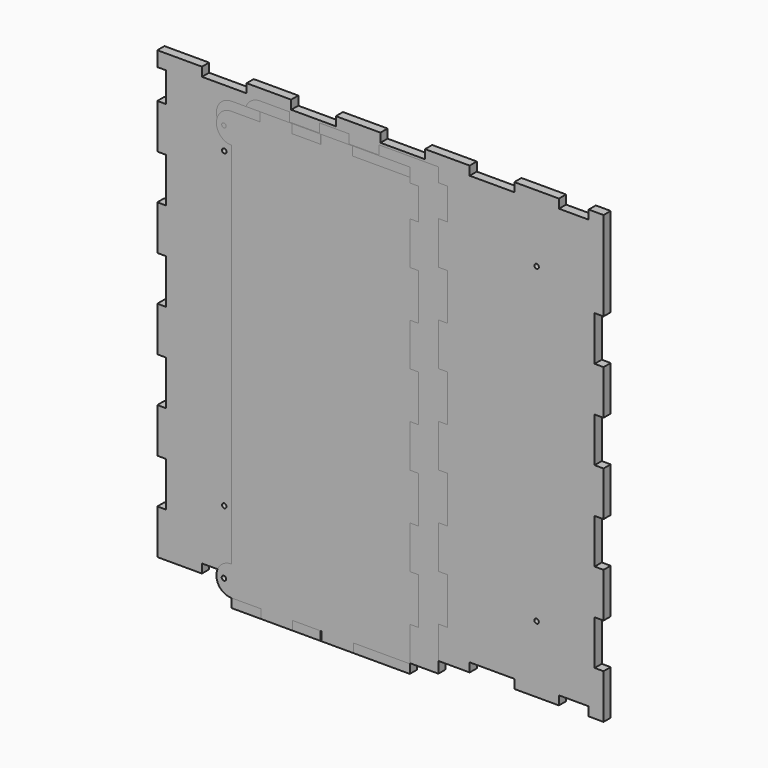
from build123d import *

# Parameters (mm, degrees)
F0_R     = 0.75
F4_DEPTH = 3
F1_R     = 0.75
F5_DEPTH = 3
F2_R     = 0.75
F6_DEPTH = 3
F3_R     = 0.75
F7_DEPTH = 3


# Not quite as in the source:
# - ends of sketch curves that miss each other by under 0.0002 mm in the source are joined


with BuildPart() as f4:
    # F0 (on Front) → F4 (new body)
    with BuildSketch(Plane.XZ):
        Polygon((-45, 72), (-60, 72), (-60, 75), (-72.0000029802, 75), (-75, 75), (-75.0000029802, 70), (-72.0000029802, 70), (-72.0000029802, 60), (-75.0000029802, 60), (-75.0000029802, 45), (-72.0000029802, 45), (-72.0000029802, 30), (-75.0000029802, 30), (-75.0000029802, 15), (-72.0000029802, 15), (-72.0000029802, 0), (-75.0000029802, 0), (-75.0000029802, -15), (-72.0000029802, -15), (-72.0000029802, -30), (-75.0000029802, -30), (-75.0000029802, -45), (-72.0000029802, -45), (-72.0000029802, -60), (-75.0000029802, -60), (-75.0000029802, -75), (-72.0000029802, -75), (-60, -75), (-60, -72), (-45, -72), (-45, -75), (-30, -75), (-30, -72), (-15, -72), (-15, -75), (0, -75), (0, -72), (15, -72), (15, -75), (30, -75), (30, -72), (45, -72), (45, -75), (60, -75), (60, -72), (70, -72), (70, -75), (75, -75), (75, -72.0000029802), (75, -60), (72, -60), (72, -45), (75, -45), (75, -30), (72, -30), (72, -15), (75, -15), (75, 0), (72, 0), (72, 15), (75, 15), (75, 30), (72, 30), (72, 45), (75, 45), (75, 60), (75, 70.000000298), (75, 75.000000298), (70, 75), (70, 72), (60, 72), (60, 75), (45, 75), (45, 72), (30, 72), (30, 75), (15, 75), (15, 72), (0, 72), (0, 75), (-15, 75), (-15, 72), (-30, 72), (-30, 75), (-45, 75), align=None)
        with Locations((-52.5, -52.5)):
            Circle(F0_R, mode=Mode.SUBTRACT)
        with Locations((52.5, -52.5)):
            Circle(F0_R, mode=Mode.SUBTRACT)
        with Locations((-52.5, 52.5)):
            Circle(F0_R, mode=Mode.SUBTRACT)
        with Locations((52.5, 52.5)):
            Circle(F0_R, mode=Mode.SUBTRACT)
    extrude(amount=F4_DEPTH)


with BuildPart() as f5:
    # F1 (on Front) → F5 (new body)
    with BuildSketch(Plane.XZ):
        with BuildLine():
            Line((22.4781758341, -64.0899424732), (22.4781758341, -63.7899424732))
            Line((22.4781758341, -63.7899424732), (22.4781758341, -48.7899424732))
            Line((22.4781758341, -48.7899424732), (22.4781758341, -48.4899424732))
            Line((22.4781758341, -48.4899424732), (19.4781758341, -48.4899424732))
            Line((19.4781758341, -48.4899424732), (19.4781758341, -34.0899424732))
            Line((19.4781758341, -34.0899424732), (22.4781758341, -34.0899424732))
            Line((22.4781758341, -34.0899424732), (22.4781758341, -33.7899424732))
            Line((22.4781758341, -33.7899424732), (22.4781758341, -18.7899424732))
            Line((22.4781758341, -18.7899424732), (22.4781758341, -18.4899424732))
            Line((22.4781758341, -18.4899424732), (19.4781758341, -18.4899424732))
            Line((19.4781758341, -18.4899424732), (19.4781758341, -4.0899424732))
            Line((19.4781758341, -4.0899424732), (22.4781758341, -4.0899424732))
            Line((22.4781758341, -4.0899424732), (22.4781758341, -3.7899424732))
            Line((22.4781758341, -3.7899424732), (22.4781758341, 11.2100575268))
            Line((22.4781758341, 11.2100575268), (22.4781758341, 11.5100575268))
            Line((22.4781758341, 11.5100575268), (19.4781758341, 11.5100575268))
            Line((19.4781758341, 11.5100575268), (19.4781758341, 25.9100575268))
            Line((19.4781758341, 25.9100575268), (22.4781758341, 25.9100575268))
            Line((22.4781758341, 25.9100575268), (22.4781758341, 26.2100575268))
            Line((22.4781758341, 26.2100575268), (22.4781758341, 41.2100575268))
            Line((22.4781758341, 41.2100575268), (22.4781758341, 41.5100575268))
            Line((22.4781758341, 41.5100575268), (19.4781758341, 41.5100575268))
            Line((19.4781758341, 41.5100575268), (19.4781758341, 55.9100575268))
            Line((19.4781758341, 55.9100575268), (22.4781758341, 55.9100567043))
            Line((22.4781758341, 55.9100567043), (22.4781758341, 56.2100567043))
            Line((22.4781758341, 56.2100567043), (22.4781758341, 66.2100567043))
            Line((22.4781758341, 66.2100567043), (22.4781758341, 66.5100567043))
            Line((22.4781758341, 66.5100567043), (19.4781758341, 66.5100567043))
            Line((19.4781758341, 66.5100567043), (19.4781758341, 71.2100575268))
            Line((19.4781758341, 71.2100575268), (-0.5218241659, 71.2100575268))
            Line((-0.5218241659, 71.2100575268), (-0.5218241659, 68.2100575268))
            Line((-0.5218241659, 68.2100575268), (-10.5218241659, 68.2100575268))
            Line((-10.5218241659, 68.2100575268), (-10.5218241659, 71.2100575268))
            Line((-10.5218241659, 71.2100575268), (-20.5218241659, 71.2100575268))
            Line((-20.5218241659, 71.2100575268), (-20.5218241659, 68.2100575268))
            Line((-20.5218241659, 68.2100575268), (-30.5218241659, 68.2100575268))
            Line((-30.5218241659, 68.2100575268), (-30.5218241659, 71.2100575268))
            Line((-30.5218241659, 71.2100575268), (-40.5218241659, 71.2100575268))
            ThreePointArc((-40.5218241659, 71.2100575268), (-45.5331626093, 66.1987190834), (-40.5218241659, 61.18738064))
            Line((-40.5218241659, 61.18738064), (-40.5218241659, -78.7899424732))
            Line((-40.5218241659, -78.7899424732), (-30.5218238408, -78.7899424732))
            Line((-30.5218238408, -78.7899424732), (-30.5218238408, -75.7899424732))
            Line((-30.5218238408, -75.7899424732), (-20.5218238408, -75.7899424732))
            Line((-20.5218238408, -75.7899424732), (-20.5218238408, -78.7899424732))
            Line((-20.5218238408, -78.7899424732), (-10.5218238408, -78.7899424732))
            Line((-10.5218238408, -78.7899424732), (-10.5218238408, -75.7899424732))
            Line((-10.5218238408, -75.7899424732), (-0.5218238408, -75.7899424732))
            Line((-0.5218238408, -75.7899424732), (-0.5218238408, -78.7899424732))
            Line((-0.5218238408, -78.7899424732), (19.4781761592, -78.7899424732))
            Line((19.4781761592, -78.7899424732), (19.4781758341, -64.0899424732))
            Line((19.4781758341, -64.0899424732), (22.4781758341, -64.0899424732))
        make_face()
        with Locations((-43.0020329712, 66.1973134672)):
            Circle(F1_R, mode=Mode.SUBTRACT)
    extrude(amount=F5_DEPTH)


with BuildPart() as f6:
    # F2 (on Front) → F6 (new body)
    with BuildSketch(Plane.XZ):
        with BuildLine():
            Line((12.8783458498, -67.2765442915), (12.8783458498, -66.9765442915))
            Line((12.8783458498, -66.9765442915), (12.8783458498, -51.9765442915))
            Line((12.8783458498, -51.9765442915), (12.8783458498, -51.6765442915))
            Line((12.8783458498, -51.6765442915), (9.8783458498, -51.6765442915))
            Line((9.8783458498, -51.6765442915), (9.8783458498, -37.2765442915))
            Line((9.8783458498, -37.2765442915), (12.8783458498, -37.2765442915))
            Line((12.8783458498, -37.2765442915), (12.8783458498, -36.9765442915))
            Line((12.8783458498, -36.9765442915), (12.8783458498, -21.9765442915))
            Line((12.8783458498, -21.9765442915), (12.8783458498, -21.6765442915))
            Line((12.8783458498, -21.6765442915), (9.8783458498, -21.6765442915))
            Line((9.8783458498, -21.6765442915), (9.8783458498, -7.2765442915))
            Line((9.8783458498, -7.2765442915), (12.8783458498, -7.2765442915))
            Line((12.8783458498, -7.2765442915), (12.8783458498, -6.9765442915))
            Line((12.8783458498, -6.9765442915), (12.8783458498, 8.0234557085))
            Line((12.8783458498, 8.0234557085), (12.8783458498, 8.3234557085))
            Line((12.8783458498, 8.3234557085), (9.8783458498, 8.3234557085))
            Line((9.8783458498, 8.3234557085), (9.8783458498, 22.7234557085))
            Line((9.8783458498, 22.7234557085), (12.8783458498, 22.7234557085))
            Line((12.8783458498, 22.7234557085), (12.8783458498, 23.0234557085))
            Line((12.8783458498, 23.0234557085), (12.8783458498, 38.0234557085))
            Line((12.8783458498, 38.0234557085), (12.8783458498, 38.3234557085))
            Line((12.8783458498, 38.3234557085), (9.8783458498, 38.3234557085))
            Line((9.8783458498, 38.3234557085), (9.8783458498, 52.7234557085))
            Line((9.8783458498, 52.7234557085), (9.8783458498, 63.3234557085))
            Line((9.8783458498, 63.3234557085), (9.8783458498, 68.0234557085))
            Line((9.8783458498, 68.0234557085), (-10.1216541502, 68.0234557085))
            Line((-10.1216541502, 68.0234557085), (-10.1216541502, 65.0234557085))
            Line((-10.1216541502, 65.0234557085), (-20.1216541502, 65.0234557085))
            Line((-20.1216541502, 65.0234557085), (-20.1216541502, 68.0234557085))
            Line((-20.1216541502, 68.0234557085), (-30.1216541502, 68.0234557085))
            Line((-30.1216541502, 68.0234557085), (-30.1216541502, 65.0234557085))
            Line((-30.1216541502, 65.0234557085), (-40.1216541502, 65.0234557085))
            Line((-40.1216541502, 65.0234557085), (-40.1216541502, 68.0234557085))
            Line((-40.1216541502, 68.0234557085), (-50.1216541502, 68.0234557085))
            ThreePointArc((-50.1216541502, 68.0234557085), (-55.1329925936, 63.0121172651), (-50.1216541502, 58.0007788217))
            Line((-50.1216541502, 58.0007788217), (-50.1216541502, -81.9765442915))
            Line((-50.1216541502, -81.9765442915), (-40.121653825, -81.9765442915))
            Line((-40.121653825, -81.9765442915), (-40.121653825, -78.9765442915))
            Line((-40.121653825, -78.9765442915), (-30.121653825, -78.9765442915))
            Line((-30.121653825, -78.9765442915), (-30.121653825, -81.9765442915))
            Line((-30.121653825, -81.9765442915), (-20.121653825, -81.9765442915))
            Line((-20.121653825, -81.9765442915), (-20.121653825, -78.9765442915))
            Line((-20.121653825, -78.9765442915), (-10.121653825, -78.9765442915))
            Line((-10.121653825, -78.9765442915), (-10.121653825, -81.9765442915))
            Line((-10.121653825, -81.9765442915), (9.878346175, -81.9765442915))
            Line((9.878346175, -81.9765442915), (9.8783458498, -67.2765442915))
            Line((9.8783458498, -67.2765442915), (12.8783458498, -67.2765442915))
        make_face()
        with Locations((-52.6018629554, 63.0107116489)):
            Circle(F2_R, mode=Mode.SUBTRACT)
    extrude(amount=F6_DEPTH)


with BuildPart() as f7:
    # F3 (on Front) → F7 (new body)
    with BuildSketch(Plane.XZ):
        with BuildLine():
            Line((12.8783458498, -67.2765442915), (12.8783458498, -66.9765442915))
            Line((12.8783458498, -66.9765442915), (12.8783458498, -51.9765442915))
            Line((12.8783458498, -51.9765442915), (12.8783458498, -51.6765442915))
            Line((12.8783458498, -51.6765442915), (9.8783458498, -51.6765442915))
            Line((9.8783458498, -51.6765442915), (9.8783458498, -37.2765442915))
            Line((9.8783458498, -37.2765442915), (12.8783458498, -37.2765442915))
            Line((12.8783458498, -37.2765442915), (12.8783458498, -36.9765442915))
            Line((12.8783458498, -36.9765442915), (12.8783458498, -21.9765442915))
            Line((12.8783458498, -21.9765442915), (12.8783458498, -21.6765442915))
            Line((12.8783458498, -21.6765442915), (9.8783458498, -21.6765442915))
            Line((9.8783458498, -21.6765442915), (9.8783458498, -7.2765442915))
            Line((9.8783458498, -7.2765442915), (12.8783458498, -7.2765442915))
            Line((12.8783458498, -7.2765442915), (12.8783458498, -6.9765442915))
            Line((12.8783458498, -6.9765442915), (12.8783458498, 8.0234557085))
            Line((12.8783458498, 8.0234557085), (12.8783458498, 8.3234557085))
            Line((12.8783458498, 8.3234557085), (9.8783458498, 8.3234557085))
            Line((9.8783458498, 8.3234557085), (9.8783458498, 22.7234557085))
            Line((9.8783458498, 22.7234557085), (12.8783458498, 22.7234557085))
            Line((12.8783458498, 22.7234557085), (12.8783458498, 23.0234557085))
            Line((12.8783458498, 23.0234557085), (12.8783458498, 38.0234557085))
            Line((12.8783458498, 38.0234557085), (12.8783458498, 38.3234557085))
            Line((12.8783458498, 38.3234557085), (9.8783458498, 38.3234557085))
            Line((9.8783458498, 38.3234557085), (9.8783458498, 52.7234557085))
            Line((9.8783458498, 52.7234557085), (12.8783458498, 52.7234557085))
            Line((12.8783458498, 52.7234557085), (12.8783458498, 53.0234557085))
            Line((12.8783458498, 53.0234557085), (12.8783458498, 63.0234557085))
            Line((12.8783458498, 63.0234557085), (12.8783458498, 63.3234557085))
            Line((12.8783458498, 63.3234557085), (9.8783458498, 63.3234557085))
            Line((9.8783458498, 63.3234557085), (9.8783458498, 65.0163069367))
            Line((9.8783458498, 65.0163069367), (-9.3813610343, 65.0163069367))
            Line((-9.3813610343, 65.0163069367), (-9.3813610343, 68.0163069367))
            Line((-9.3813610343, 68.0163069367), (-20.0216541528, 68.0163069367))
            Line((-20.0216541528, 68.0163069367), (-20.0216541528, 65.0163069367))
            Line((-20.0216541528, 65.0163069367), (-20.1232303983, 65.0163069367))
            Line((-20.1232303983, 65.0163069367), (-20.1235094473, 65.0163069367))
            Line((-20.1235094473, 65.0163069367), (-29.8016541528, 65.0163069367))
            Line((-29.8016541528, 65.0163069367), (-29.8016541528, 68.0163069367))
            Line((-29.8016541528, 68.0163069367), (-30.1216541528, 68.0163069367))
            Line((-30.1216541528, 68.0163069367), (-30.4416541528, 68.0163069367))
            Line((-30.4416541528, 68.0163069367), (-40.4416541528, 68.0163069367))
            Line((-40.4416541528, 68.0163069367), (-40.4416541528, 65.0163069367))
            Line((-40.4416541528, 65.0163069367), (-50.1216541502, 65.0163069367))
            Line((-50.1216541502, 65.0163069367), (-50.3889447089, 65.0163069367))
            ThreePointArc((-50.3889447089, 65.0163069367), (-55.131208942, 59.8784089661), (-50.1216541502, 55.0007633865))
            Line((-50.1216541502, 55.0007633865), (-50.1216541502, -68.9538648708))
            ThreePointArc((-50.1216541502, -68.9538648708), (-55.1329925936, -73.9652033142), (-50.1216541502, -78.9765417576))
            Line((-50.1216541502, -78.9765417576), (-49.8543635914, -78.9765417576))
            Line((-49.8543635914, -78.9765417576), (-40.1743635941, -78.9765417576))
            Line((-40.1743635941, -78.9765417576), (-40.1743635941, -81.9765417576))
            Line((-40.1743635941, -81.9765417576), (-30.1743635941, -81.9765417576))
            Line((-30.1743635941, -81.9765417576), (-29.8543635941, -81.9765417576))
            Line((-29.8543635941, -81.9765417576), (-29.5343635941, -81.9765417576))
            Line((-29.5343635941, -81.9765417576), (-29.5343635941, -78.9765417576))
            Line((-29.5343635941, -78.9765417576), (-19.8562188886, -78.9765417576))
            Line((-19.8562188886, -78.9765417576), (-19.8559398396, -78.9765417576))
            Line((-19.8559398396, -78.9765417576), (-19.7543635941, -78.9765417576))
            Line((-19.7543635941, -78.9765417576), (-19.7543635941, -81.9765417576))
            Line((-19.7543635941, -81.9765417576), (-9.1140704756, -81.9765417576))
            Line((-9.1140704756, -81.9765417576), (-9.1140704756, -78.9765417578))
            Line((-9.1140704756, -78.9765417578), (9.8783458498, -78.9765417581))
            Line((9.8783458498, -78.9765417576), (9.8783458498, -67.2765442915))
            Line((9.8783458498, -67.2765442915), (12.8783458498, -67.2765442915))
        make_face()
        with Locations((-52.6018629554, -73.9666089304)):
            Circle(F3_R, mode=Mode.SUBTRACT)
        with Locations((-52.6018626303, 60.0106962137)):
            Circle(F3_R, mode=Mode.SUBTRACT)
    extrude(amount=F7_DEPTH)


solid = Compound([f4.part, f5.part, f6.part, f7.part])
